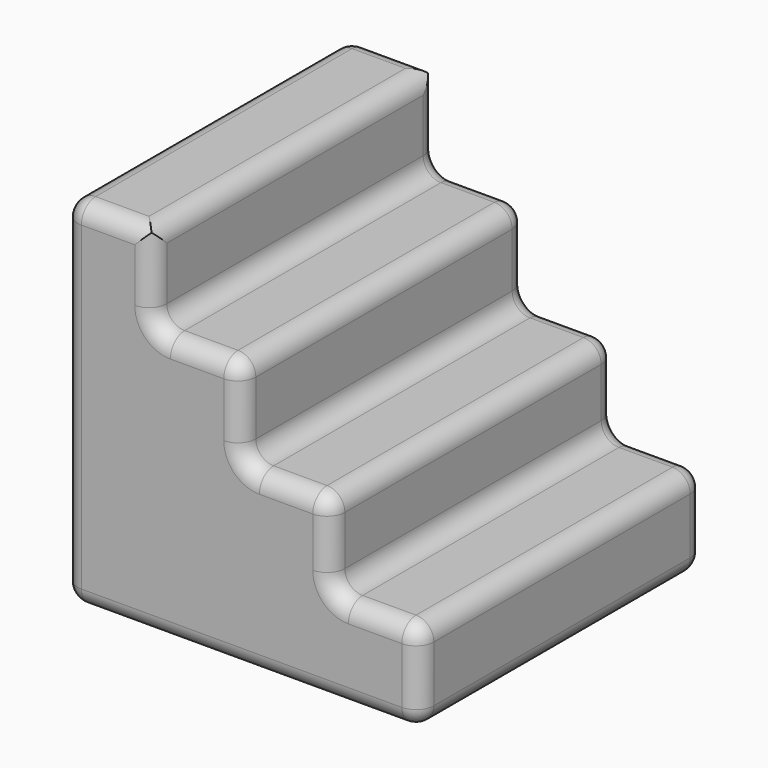
from build123d import *

# Parameters (mm, degrees)
F0_W         = 100
F0_H         = 100
F1_DEPTH     = 100
F3_DEPTH     = 107.7
F4_F1_R      = 5
F4_F2_R      = 5
F5_T1_DEPTH  = 100
F5_T3_DEPTH  = 27.5
F5_T5_DEPTH  = 90
F5_T7_DEPTH  = 125
F5_T9_DEPTH  = 33.2688637823
F5_T11_DEPTH = 90
F5_T13_DEPTH = 90
F5_S17_W     = 5.1
F5_S17_H     = 5.1
F5_T18_DEPTH = 5.1
F5_S23_W     = 5.1
F5_S23_H     = 5.1
F5_T24_DEPTH = 5.1
F5_S29_W     = 5.1
F5_S29_H     = 5.1
F5_T30_DEPTH = 5.1
F5_S35_W     = 5.1
F5_S35_H     = 5.1
F5_T36_DEPTH = 5.1
F5_S41_W     = 5.1
F5_S41_H     = 5.1
F5_T42_DEPTH = 5.1
F5_S47_W     = 5.1
F5_S47_H     = 5.1
F5_T48_DEPTH = 5.1
F5_T51_DEPTH = 15.3089666367
F5_T53_DEPTH = 90
F5_T55_DEPTH = 13.9221695811
F5_T57_DEPTH = 15
F5_T59_DEPTH = 15
F5_S63_W     = 5.1
F5_S63_H     = 5.1
F5_T64_DEPTH = 5.1
F5_S69_W     = 5.1
F5_S69_H     = 5.1
F5_T70_DEPTH = 5.1
F5_T74_ANGLE = 90
F5_T76_ANGLE = 90
F5_T78_ANGLE = 90
F5_T80_ANGLE = 90
F5_T82_ANGLE = 90
F5_T84_ANGLE = 90
F5_T86_ANGLE = 90
F5_T88_ANGLE = 90


# Not quite as in the source:
# - a fillet or chamfer that OpenCascade refuses, or shapes differently, is made with other operations: its cross-section is extruded or revolved along the edge and cut away or added


with BuildPart() as f1:
    # F0 (on Top) → F1 (new body)
    with BuildSketch(Plane.XY):
        with Locations((50, 50)):
            Rectangle(F0_W, F0_H)
    extrude(amount=F1_DEPTH)

    # F2 (on face) → F3 (cut)
    with BuildSketch(Plane.XZ):
        Polygon((100, 100), (25, 100), (25, 75), (50, 75), (50, 49.6910333633), (75, 49.6910333633), (75, 25.7688637823), (100, 25.7688637823), align=None)
    extrude(amount=-F3_DEPTH, mode=Mode.SUBTRACT)

    # F4: fillet of radius 5 on 4 edges, made by hand

    # F4_f1
    f4_f1_edges = [f1.edges().sort_by_distance(p)[0] for p in [
        (25, 50, 75),
    ]]
    fillet(f4_f1_edges, radius=F4_F1_R)

    # F4_f2
    f4_f2_edges = [f1.edges().sort_by_distance(p)[0] for p in [
        (25, 0, 90),
        (25, 100, 90),
        (25, 50, 100),
        (26.4644660941, 100, 76.4644660941),
        (26.4644660941, 0, 76.4644660941),
    ]]
    fillet(f4_f2_edges, radius=F4_F2_R)

    # F5: fillet of radius 5 on 33 edges, made by hand

    # F5_s2 → F5_t1 (join)
    with BuildSketch(Plane.XZ.offset(-100)):
        with BuildLine():
            ThreePointArc((50, 54.6910333633), (51.4644660941, 51.1554994574), (55, 49.6910333633))
            Line((55, 49.6910333633), (50, 49.6910333633))
            Line((50, 49.6910333633), (50, 54.6910333633))
        make_face()
        with BuildLine():
            ThreePointArc((80, 25.7688637823), (76.4644660941, 27.2333298764), (75, 30.7688637823))
            Line((75, 30.7688637823), (75, 25.7688637823))
            Line((75, 25.7688637823), (80, 25.7688637823))
        make_face()
    extrude(amount=F5_T1_DEPTH)

    # F5_s4 → F5_t3 (cut)
    with BuildSketch(Plane.YZ.offset(5)):
        with BuildLine():
            ThreePointArc((100, 95), (98.5355339059, 98.5355339059), (95, 100))
            Line((95, 100), (100, 100))
            Line((100, 100), (100, 95))
        make_face()
        with BuildLine():
            ThreePointArc((5, 100), (1.4644660941, 98.5355339059), (0, 95))
            Line((0, 95), (0, 100))
            Line((0, 100), (5, 100))
        make_face()
    extrude(amount=F5_T3_DEPTH, mode=Mode.SUBTRACT)

    # F5_s6 → F5_t5 (cut)
    with BuildSketch(Plane.XZ.offset(-95)):
        with BuildLine():
            ThreePointArc((5, 100), (1.4644660941, 98.5355339059), (0, 95))
            Line((0, 95), (0, 100))
            Line((0, 100), (5, 100))
        make_face()
        with BuildLine():
            ThreePointArc((95, 0), (98.5355339059, 1.4644660941), (100, 5))
            Line((100, 5), (100, 0))
            Line((100, 0), (95, 0))
        make_face()
        with BuildLine():
            ThreePointArc((0, 5), (1.4644660941, 1.4644660941), (5, 0))
            Line((5, 0), (0, 0))
            Line((0, 0), (0, 5))
        make_face()
    extrude(amount=F5_T5_DEPTH, mode=Mode.SUBTRACT)

    # F5_s8 → F5_t7 (cut)
    with BuildSketch(Plane.XZ.offset(-112.5)):
        with BuildLine():
            ThreePointArc((70, 49.6910333633), (73.5355339059, 48.2265672693), (75, 44.6910333633))
            Line((75, 44.6910333633), (75, 49.6910333633))
            Line((75, 49.6910333633), (70, 49.6910333633))
        make_face()
        with BuildLine():
            ThreePointArc((100, 20.7688637823), (98.5355339059, 24.3043976882), (95, 25.7688637823))
            Line((95, 25.7688637823), (100, 25.7688637823))
            Line((100, 25.7688637823), (100, 20.7688637823))
        make_face()
    extrude(amount=F5_T7_DEPTH, mode=Mode.SUBTRACT)

    # F5_s10 → F5_t9 (cut)
    with BuildSketch(Plane.XY.offset(5)):
        with BuildLine():
            ThreePointArc((95, 100), (98.5355339059, 98.5355339059), (100, 95))
            Line((100, 95), (100, 100))
            Line((100, 100), (95, 100))
        make_face()
        with BuildLine():
            ThreePointArc((100, 5), (98.5355339059, 1.4644660941), (95, 0))
            Line((95, 0), (100, 0))
            Line((100, 0), (100, 5))
        make_face()
    extrude(amount=F5_T9_DEPTH, mode=Mode.SUBTRACT)

    # F5_s12 → F5_t11 (cut)
    with BuildSketch(Plane.XY.offset(5)):
        with BuildLine():
            ThreePointArc((0, 5), (1.4644660941, 1.4644660941), (5, 0))
            Line((5, 0), (0, 0))
            Line((0, 0), (0, 5))
        make_face()
        with BuildLine():
            ThreePointArc((5, 100), (1.4644660941, 98.5355339059), (0, 95))
            Line((0, 95), (0, 100))
            Line((0, 100), (5, 100))
        make_face()
    extrude(amount=F5_T11_DEPTH, mode=Mode.SUBTRACT)

    # F5_s14 → F5_t13 (cut)
    with BuildSketch(Plane.YZ.offset(5)):
        with BuildLine():
            ThreePointArc((5, 0), (1.4644660941, 1.4644660941), (0, 5))
            Line((0, 5), (0, 0))
            Line((0, 0), (5, 0))
        make_face()
        with BuildLine():
            ThreePointArc((100, 5), (98.5355339059, 1.4644660941), (95, 0))
            Line((95, 0), (100, 0))
            Line((100, 0), (100, 5))
        make_face()
    extrude(amount=F5_T13_DEPTH, mode=Mode.SUBTRACT)


with BuildPart() as f5_tool16:
    # F5_s17 → F5_t18 (new body)
    with BuildSketch(Plane.XZ.offset(-95)):
        with Locations((2.45, 97.55)):
            Rectangle(F5_S17_W, F5_S17_H)
    extrude(amount=-F5_T18_DEPTH)

    # F5_s19 → F5_t20 (revolve, cut)
    with BuildSketch(Plane(origin=(5, 95, 95), x_dir=(0.7071067812, 0, -0.7071067812), z_dir=(0.7071067812, 0, 0.7071067812))):
        with BuildLine():
            ThreePointArc((0, -5), (5, 0), (0, 5))
            Line((0, 5), (0, -5))
        make_face()
    revolve(axis=Axis((5, 95, 95), (0, 1, 0)), mode=Mode.SUBTRACT)


with BuildPart() as f1_1:
    add(f1.part)

    # F5_t15: cut F5_tool16
    add(f5_tool16.part, mode=Mode.SUBTRACT)


with BuildPart() as f5_tool22:
    # F5_s23 → F5_t24 (new body)
    with BuildSketch(Plane.XY.offset(95)):
        with Locations((2.45, 2.45)):
            Rectangle(F5_S23_W, F5_S23_H)
    extrude(amount=F5_T24_DEPTH)

    # F5_s25 → F5_t26 (revolve, cut)
    with BuildSketch(Plane(origin=(5, 5, 95), x_dir=(0.7071067812, 0.7071067812, 0), z_dir=(0.7071067812, -0.7071067812, 0))):
        with BuildLine():
            ThreePointArc((0, -5), (5, 0), (0, 5))
            Line((0, 5), (0, -5))
        make_face()
    revolve(axis=Axis((5, 5, 95), (0, 0, 1)), mode=Mode.SUBTRACT)


with BuildPart() as f1_2:
    add(f1_1.part)

    # F5_t21: cut F5_tool22
    add(f5_tool22.part, mode=Mode.SUBTRACT)


with BuildPart() as f5_tool28:
    # F5_s29 → F5_t30 (new body)
    with BuildSketch(Plane.XZ.offset(-5)):
        with Locations((97.55, 2.45)):
            Rectangle(F5_S29_W, F5_S29_H)
    extrude(amount=F5_T30_DEPTH)

    # F5_s31 → F5_t32 (revolve, cut)
    with BuildSketch(Plane(origin=(95, 5, 5), x_dir=(-0.7071067812, 0, 0.7071067812), z_dir=(0.7071067812, 0, 0.7071067812))):
        with BuildLine():
            ThreePointArc((0, -5), (5, 0), (0, 5))
            Line((0, 5), (0, -5))
        make_face()
    revolve(axis=Axis((95, 5, 5), (0, -1, 0)), mode=Mode.SUBTRACT)


with BuildPart() as f1_3:
    add(f1_2.part)

    # F5_t27: cut F5_tool28
    add(f5_tool28.part, mode=Mode.SUBTRACT)


with BuildPart() as f5_tool34:
    # F5_s35 → F5_t36 (new body)
    with BuildSketch(Plane.XZ.offset(-95)):
        with Locations((97.55, 2.45)):
            Rectangle(F5_S35_W, F5_S35_H)
    extrude(amount=-F5_T36_DEPTH)

    # F5_s37 → F5_t38 (revolve, cut)
    with BuildSketch(Plane(origin=(95, 95, 5), x_dir=(-0.7071067812, 0, 0.7071067812), z_dir=(-0.7071067812, 0, -0.7071067812))):
        with BuildLine():
            ThreePointArc((0, -5), (5, 0), (0, 5))
            Line((0, 5), (0, -5))
        make_face()
    revolve(axis=Axis((95, 95, 5), (0, 1, 0)), mode=Mode.SUBTRACT)


with BuildPart() as f1_4:
    add(f1_3.part)

    # F5_t33: cut F5_tool34
    add(f5_tool34.part, mode=Mode.SUBTRACT)


with BuildPart() as f5_tool40:
    # F5_s41 → F5_t42 (new body)
    with BuildSketch(Plane.XY.offset(5)):
        with Locations((2.45, 2.45)):
            Rectangle(F5_S41_W, F5_S41_H)
    extrude(amount=-F5_T42_DEPTH)

    # F5_s43 → F5_t44 (revolve, cut)
    with BuildSketch(Plane(origin=(5, 5, 5), x_dir=(0.7071067812, 0.7071067812, 0), z_dir=(-0.7071067812, 0.7071067812, 0))):
        with BuildLine():
            ThreePointArc((0, -5), (5, 0), (0, 5))
            Line((0, 5), (0, -5))
        make_face()
    revolve(axis=Axis((5, 5, 5), (0, 0, -1)), mode=Mode.SUBTRACT)


with BuildPart() as f1_5:
    add(f1_4.part)

    # F5_t39: cut F5_tool40
    add(f5_tool40.part, mode=Mode.SUBTRACT)


with BuildPart() as f5_tool46:
    # F5_s47 → F5_t48 (new body)
    with BuildSketch(Plane.XZ.offset(-95)):
        with Locations((2.45, 2.45)):
            Rectangle(F5_S47_W, F5_S47_H)
    extrude(amount=-F5_T48_DEPTH)

    # F5_s49 → F5_t50 (revolve, cut)
    with BuildSketch(Plane(origin=(5, 95, 5), x_dir=(0.7071067812, 0, 0.7071067812), z_dir=(-0.7071067812, 0, 0.7071067812))):
        with BuildLine():
            ThreePointArc((0, -5), (5, 0), (0, 5))
            Line((0, 5), (0, -5))
        make_face()
    revolve(axis=Axis((5, 95, 5), (0, 1, 0)), mode=Mode.SUBTRACT)


with BuildPart() as f1_6:
    add(f1_5.part)

    # F5_t45: cut F5_tool46
    add(f5_tool46.part, mode=Mode.SUBTRACT)

    # F5_s52 → F5_t51 (cut)
    with BuildSketch(Plane.XY.offset(54.6910333633)):
        with BuildLine():
            ThreePointArc((50, 5), (48.5355339059, 1.4644660941), (45, 0))
            Line((45, 0), (50, 0))
            Line((50, 0), (50, 5))
        make_face()
        with BuildLine():
            ThreePointArc((45, 100), (48.5355339059, 98.5355339059), (50, 95))
            Line((50, 95), (50, 100))
            Line((50, 100), (45, 100))
        make_face()
    extrude(amount=F5_T51_DEPTH, mode=Mode.SUBTRACT)

    # F5_s54 → F5_t53 (cut)
    with BuildSketch(Plane.XZ.offset(-95)):
        with BuildLine():
            ThreePointArc((50, 70), (48.5355339059, 73.5355339059), (45, 75))
            Line((45, 75), (50, 75))
            Line((50, 75), (50, 70))
        make_face()
    extrude(amount=F5_T53_DEPTH, mode=Mode.SUBTRACT)

    # F5_s56 → F5_t55 (cut)
    with BuildSketch(Plane.XY.offset(30.7688637823)):
        with BuildLine():
            ThreePointArc((75, 5), (73.5355339059, 1.4644660941), (70, 0))
            Line((70, 0), (75, 0))
            Line((75, 0), (75, 5))
        make_face()
        with BuildLine():
            ThreePointArc((70, 100), (73.5355339059, 98.5355339059), (75, 95))
            Line((75, 95), (75, 100))
            Line((75, 100), (70, 100))
        make_face()
    extrude(amount=F5_T55_DEPTH, mode=Mode.SUBTRACT)

    # F5_s58 → F5_t57 (cut)
    with BuildSketch(Plane.YZ.offset(55)):
        with BuildLine():
            ThreePointArc((5, 49.6910333633), (1.4644660941, 48.2265672693), (0, 44.6910333633))
            Line((0, 44.6910333633), (0, 49.6910333633))
            Line((0, 49.6910333633), (5, 49.6910333633))
        make_face()
        with BuildLine():
            ThreePointArc((100, 44.6910333633), (98.5355339059, 48.2265672693), (95, 49.6910333633))
            Line((95, 49.6910333633), (100, 49.6910333633))
            Line((100, 49.6910333633), (100, 44.6910333633))
        make_face()
    extrude(amount=F5_T57_DEPTH, mode=Mode.SUBTRACT)

    # F5_s60 → F5_t59 (cut)
    with BuildSketch(Plane.YZ.offset(80)):
        with BuildLine():
            ThreePointArc((5, 25.7688637823), (1.4644660941, 24.3043976882), (0, 20.7688637823))
            Line((0, 20.7688637823), (0, 25.7688637823))
            Line((0, 25.7688637823), (5, 25.7688637823))
        make_face()
        with BuildLine():
            ThreePointArc((100, 20.7688637823), (98.5355339059, 24.3043976882), (95, 25.7688637823))
            Line((95, 25.7688637823), (100, 25.7688637823))
            Line((100, 25.7688637823), (100, 20.7688637823))
        make_face()
    extrude(amount=F5_T59_DEPTH, mode=Mode.SUBTRACT)


with BuildPart() as f5_tool62:
    # F5_s63 → F5_t64 (new body)
    with BuildSketch(Plane.XZ.offset(-95)):
        with Locations((97.55, 23.3188637823)):
            Rectangle(F5_S63_W, F5_S63_H)
    extrude(amount=-F5_T64_DEPTH)

    # F5_s65 → F5_t66 (revolve, cut)
    with BuildSketch(Plane(origin=(95, 95, 20.7688637823), x_dir=(-0.7071067812, 0, -0.7071067812), z_dir=(0.7071067812, 0, -0.7071067812))):
        with BuildLine():
            ThreePointArc((0, -5), (5, 0), (0, 5))
            Line((0, 5), (0, -5))
        make_face()
    revolve(axis=Axis((95, 95, 20.7688637823), (0, 1, 0)), mode=Mode.SUBTRACT)


with BuildPart() as f1_7:
    add(f1_6.part)

    # F5_t61: cut F5_tool62
    add(f5_tool62.part, mode=Mode.SUBTRACT)


with BuildPart() as f5_tool68:
    # F5_s69 → F5_t70 (new body)
    with BuildSketch(Plane.XY.offset(20.7688637823)):
        with Locations((97.55, 2.45)):
            Rectangle(F5_S69_W, F5_S69_H)
    extrude(amount=F5_T70_DEPTH)

    # F5_s71 → F5_t72 (revolve, cut)
    with BuildSketch(Plane(origin=(95, 5, 20.7688637823), x_dir=(-0.7071067812, 0.7071067812, 0), z_dir=(0.7071067812, 0.7071067812, 0))):
        with BuildLine():
            ThreePointArc((0, -5), (5, 0), (0, 5))
            Line((0, 5), (0, -5))
        make_face()
    revolve(axis=Axis((95, 5, 20.7688637823), (0, 0, 1)), mode=Mode.SUBTRACT)


with BuildPart() as f1_8:
    add(f1_7.part)

    # F5_t67: cut F5_tool68
    add(f5_tool68.part, mode=Mode.SUBTRACT)

    # F5_s73 → F5_t74 (revolve, cut)
    with BuildSketch(Plane.XZ.offset(-5)):
        with BuildLine():
            ThreePointArc((50, 70), (48.5355339059, 73.5355339059), (45, 75))
            Line((45, 75), (50, 75))
            Line((50, 75), (50, 70))
        make_face()
    revolve(axis=Axis((50, 5, 70), (1, 0, 0)), revolution_arc=F5_T74_ANGLE, mode=Mode.SUBTRACT)

    # F5_s75 → F5_t76 (revolve, cut)
    with BuildSketch(Plane.XY.offset(70)):
        with BuildLine():
            ThreePointArc((45, 100), (48.5355339059, 98.5355339059), (50, 95))
            Line((50, 95), (50, 100))
            Line((50, 100), (45, 100))
        make_face()
    revolve(axis=Axis((50, 95, 70), (1, 0, 0)), revolution_arc=F5_T76_ANGLE, mode=Mode.SUBTRACT)

    # F5_s77 → F5_t78 (revolve, cut)
    with BuildSketch(Plane.XY.offset(54.6910333633)):
        with BuildLine():
            ThreePointArc((45, 100), (48.5355339059, 98.5355339059), (50, 95))
            Line((50, 95), (50, 100))
            Line((50, 100), (45, 100))
        make_face()
    revolve(axis=Axis((55, 100, 54.6910333633), (0, -1, 0)), revolution_arc=F5_T78_ANGLE, mode=Mode.SUBTRACT)

    # F5_s79 → F5_t80 (revolve, cut)
    with BuildSketch(Plane.XY.offset(44.6910333633)):
        with BuildLine():
            ThreePointArc((70, 100), (73.5355339059, 98.5355339059), (75, 95))
            Line((75, 95), (75, 100))
            Line((75, 100), (70, 100))
        make_face()
    revolve(axis=Axis((70, 100, 44.6910333633), (0, -1, 0)), revolution_arc=F5_T80_ANGLE, mode=Mode.SUBTRACT)

    # F5_s81 → F5_t82 (revolve, cut)
    with BuildSketch(Plane.YZ.offset(80)):
        with BuildLine():
            ThreePointArc((100, 20.7688637823), (98.5355339059, 24.3043976882), (95, 25.7688637823))
            Line((95, 25.7688637823), (100, 25.7688637823))
            Line((100, 25.7688637823), (100, 20.7688637823))
        make_face()
    revolve(axis=Axis((80, 100, 30.7688637823), (0, 1, 0)), revolution_arc=F5_T82_ANGLE, mode=Mode.SUBTRACT)

    # F5_s83 → F5_t84 (revolve, cut)
    with BuildSketch(Plane.YZ.offset(80)):
        with BuildLine():
            ThreePointArc((5, 25.7688637823), (1.4644660941, 24.3043976882), (0, 20.7688637823))
            Line((0, 20.7688637823), (0, 25.7688637823))
            Line((0, 25.7688637823), (5, 25.7688637823))
        make_face()
    revolve(axis=Axis((80, 0, 30.7688637823), (0, 1, 0)), revolution_arc=F5_T84_ANGLE, mode=Mode.SUBTRACT)

    # F5_s85 → F5_t86 (revolve, cut)
    with BuildSketch(Plane.XY.offset(54.6910333633)):
        with BuildLine():
            ThreePointArc((50, 5), (48.5355339059, 1.4644660941), (45, 0))
            Line((45, 0), (50, 0))
            Line((50, 0), (50, 5))
        make_face()
    revolve(axis=Axis((55, 0, 54.6910333633), (0, -1, 0)), revolution_arc=F5_T86_ANGLE, mode=Mode.SUBTRACT)

    # F5_s87 → F5_t88 (revolve, cut)
    with BuildSketch(Plane.XY.offset(44.6910333633)):
        with BuildLine():
            ThreePointArc((75, 5), (73.5355339059, 1.4644660941), (70, 0))
            Line((70, 0), (75, 0))
            Line((75, 0), (75, 5))
        make_face()
    revolve(axis=Axis((70, 0, 44.6910333633), (0, -1, 0)), revolution_arc=F5_T88_ANGLE, mode=Mode.SUBTRACT)


solid = f1_8.part
